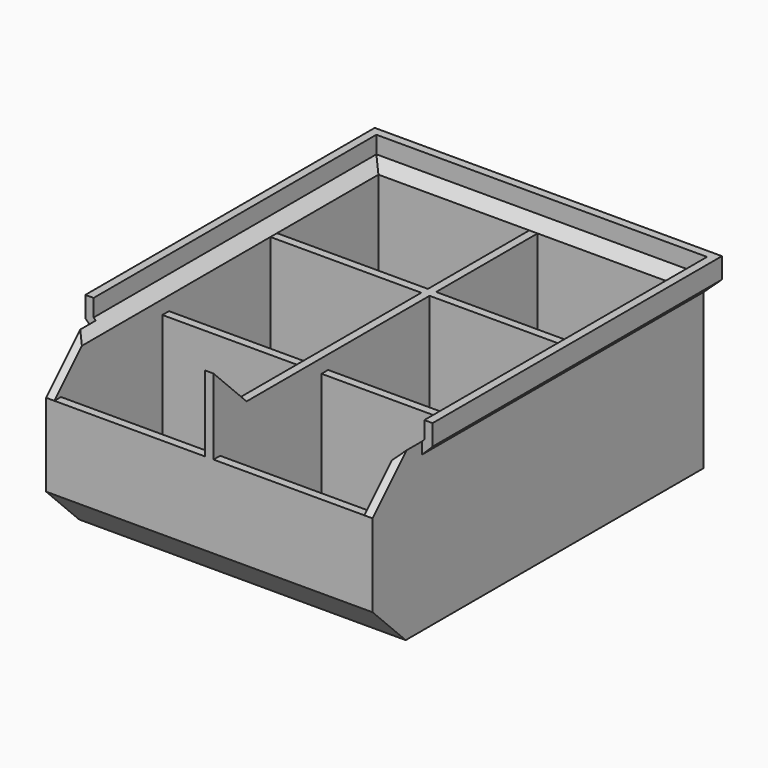
from build123d import *

# Parameters (mm, degrees)
F1_DEPTH  = 2
F2_W      = 2
F2_H      = 33
F2_H_2    = 38
F3_DEPTH  = 75
F5_DEPTH  = 2
F6_W      = 2.5
F6_H      = 87.5
F7_DEPTH  = 7.5
F9_DEPTH  = 102.501
F11_DEPTH = 84.001
F13_DEPTH = 98
F15_DEPTH = 2.5
F17_DEPTH = 2.5
F19_DEPTH = 2.5
F21_DEPTH = 2.5
F23_W     = 30.666666667
F23_H     = 0.8284271247
F23_W_2   = 30.6666666667
F23_H_2   = 35.5
F24_DEPTH = 2


# Not quite as in the source:
# - a feature names something its author has since deleted; it is built from what else it names


with BuildPart() as f1:
    # F0 (on Right) → F1 (new body)
    with BuildSketch(Plane.YZ):
        Polygon((0, 10), (10, 0), (100, 0), (100, 37.5), (100, 45), (15, 45), (0, 30), align=None)
        Polygon((100, 45), (100, 37.5), (102.5, 40), (102.5, 45), align=None)
    extrude(amount=-F1_DEPTH)

    # F2 (on face) → F3 (join)
    with BuildSketch(Plane.YZ):
        Polygon((2, 30), (0, 30), (0, 10), (10, 0), (100, 0), (100, 37.5), (102.5, 40), (102.5, 45), (100.5, 45), (100.5, 40.8284271247), (98, 38.3284271247), (98, 2), (67.3333333333, 2), (65.3333333333, 2), (34.6666666667, 2), (32.6666666667, 2), (10.8284271247, 2), (2, 10.8284271247), align=None)
        with Locations((33.6666666667, 18.5)):
            Rectangle(F2_W, F2_H)
        with Locations((66.3333333333, 21)):
            Rectangle(F2_W, F2_H_2)
    extrude(amount=F3_DEPTH)

    # F4 (on face) → F5 (join)
    with BuildSketch(Plane.YZ.offset(75)):
        Polygon((100.5, 45), (15, 45), (0, 30), (0, 10), (10, 0), (100, 0), (100, 37.5), (102.5, 40), (102.5, 45), align=None)
    extrude(amount=F5_DEPTH)

    # F6 (on face) → F7 (join)
    with BuildSketch(Plane.XY.offset(45)):
        with Locations((-3.25, 58.75)):
            Rectangle(F6_W, F6_H)
        with Locations((78.25, 58.75)):
            Rectangle(F6_W, F6_H)
    extrude(amount=-F7_DEPTH)

    # F8 (on face) → F9 (cut, through all)
    with BuildSketch(Plane(origin=(0, 102.5, 0), x_dir=(-1, 0, 0), z_dir=(0, 1, 0))):
        Polygon((-79.5, 37.5), (-77, 37.5), (-79.5, 40), align=None)
        Polygon((4.5, 40), (2, 37.5), (4.5, 37.5), align=None)
    extrude(amount=-F9_DEPTH, mode=Mode.SUBTRACT)

    # F10 (on face) → F11 (cut, through all)
    with BuildSketch(Plane.YZ.offset(79.5)):
        Polygon((100, 37.5), (102.5, 37.5), (102.5, 40), align=None)
    extrude(amount=-F11_DEPTH, mode=Mode.SUBTRACT)

    # F12 (on face) → F13 (cut, through all)
    with BuildSketch(Plane.XZ):
        Polygon((77, 45), (75, 45), (0, 45), (-2, 45), (-2.5, 45), (-2.5, 40.8284271247), (0, 38.3284271247), (75, 38.3284271247), (75.3564065228, 38.6848336475), (77.5, 40.8284271247), (77.5, 45), align=None)
    extrude(amount=-F13_DEPTH, mode=Mode.SUBTRACT)

    # F14 (on face) → F15 (cut, through all)
    with BuildSketch(Plane(origin=(75, 0, 0), x_dir=(0, -1, 0), z_dir=(-1, 0, 0))):
        Polygon((-100.5, 40.8284271247), (-98, 38.3284271247), (-98, 45), (-100.5, 45), align=None)
    extrude(amount=-F15_DEPTH, mode=Mode.SUBTRACT)

    # F16 (on face) → F17 (join, through all)
    with BuildSketch(Plane(origin=(0, 98, 0), x_dir=(-1, 0, 0), z_dir=(0, 1, 0))):
        Polygon((-77.5, 38.3284271247), (-75, 38.3284271247), (-77.5, 40.8284271247), align=None)
    extrude(amount=F17_DEPTH)

    # F18 (on face) → F19 (cut, through all)
    with BuildSketch(Plane.YZ):
        Polygon((100.5, 40.8284271247), (100.5, 45), (98, 45), (98, 38.3284271247), align=None)
    extrude(amount=-F19_DEPTH, mode=Mode.SUBTRACT)

    # F20 (on face) → F21 (join, through all)
    with BuildSketch(Plane(origin=(0, 98, 0), x_dir=(-1, 0, 0), z_dir=(0, 1, 0))):
        Polygon((2.5, 38.3284271247), (2.5, 40.8284271247), (0, 38.3284271247), align=None)
    extrude(amount=F21_DEPTH)

    # F23 (on offset) → F24 (join)
    with BuildSketch(Plane.YZ.offset(36.5)):
        with Locations((82.6666666668, 37.9142135624)):
            Rectangle(F23_W, F23_H)
        with Locations((82.6666666667, 19.75)):
            Rectangle(F23_W_2, F23_H_2)
        Polygon((65.3333333333, 2), (65.3333333333, 37.5), (65.3333333333, 38.3284271247), (10, 38.3284271247), (10, 2.8284271247), (10.8284271247, 2), (32.6666666667, 2), (32.6666666667, 35), (34.6666666667, 35), (34.6666666667, 2), align=None)
        Polygon((10, 2.8284271247), (10, 38.3284271247), (2, 30), (2, 10.8284271247), align=None)
        Polygon((0, 30), (8.3284271248, 38.3284271248), (9.1642135624, 39.1642135624), (0, 48.3284271247), align=None)
        Polygon((2, 30), (10, 38.3284271247), (8.3284271251, 38.3284271247), (0, 30), align=None)
        Polygon((8.3284271251, 38.3284271247), (10, 38.3284271247), (9.1642135624, 39.1642135624), align=None)
    extrude(amount=F24_DEPTH)


solid = f1.part
